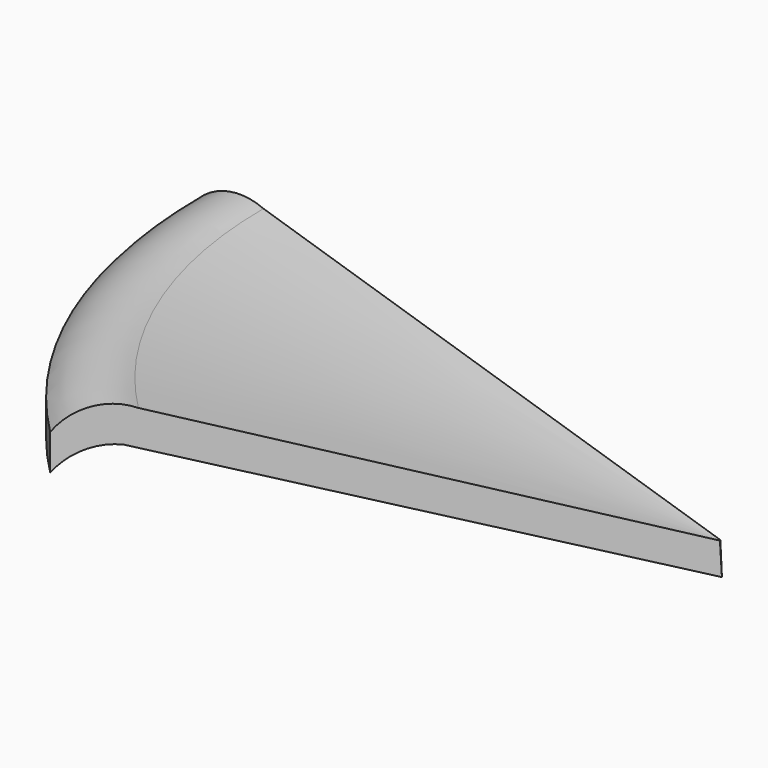
from build123d import *

# Parameters (mm, degrees)
F1_ANGLE = 45


# Not quite as in the source:
# - a feature names something its author has since deleted; it is built from what else it names


with BuildPart() as f1:
    # F0 (on Front) → F1 (revolve)
    with BuildSketch(Plane.XZ):
        with BuildLine():
            Line((0, 0), (-0.3200573587, 6.5955988818))
            Line((-0.3200573587, 6.5955988818), (-93.7548232766, 35.8510324721))
            ThreePointArc((-93.7548232766, 35.8510324721), (-101.4397958576, 36.5208008084), (-107.92452842, 32.3428064585))
            Line((-107.92452842, 32.3428064585), (-107.92452842, 24.9973144382))
            ThreePointArc((-107.92452842, 24.9973144382), (-102.6379346155, 28.7570956855), (-96.1832379704, 29.4058793942))
            Line((-96.1832379704, 29.4058793942), (0, 0))
        make_face()
    revolve(axis=Axis((0, 0, 59.7953810357), (0, 0, 1)), revolution_arc=F1_ANGLE)


solid = f1.part
